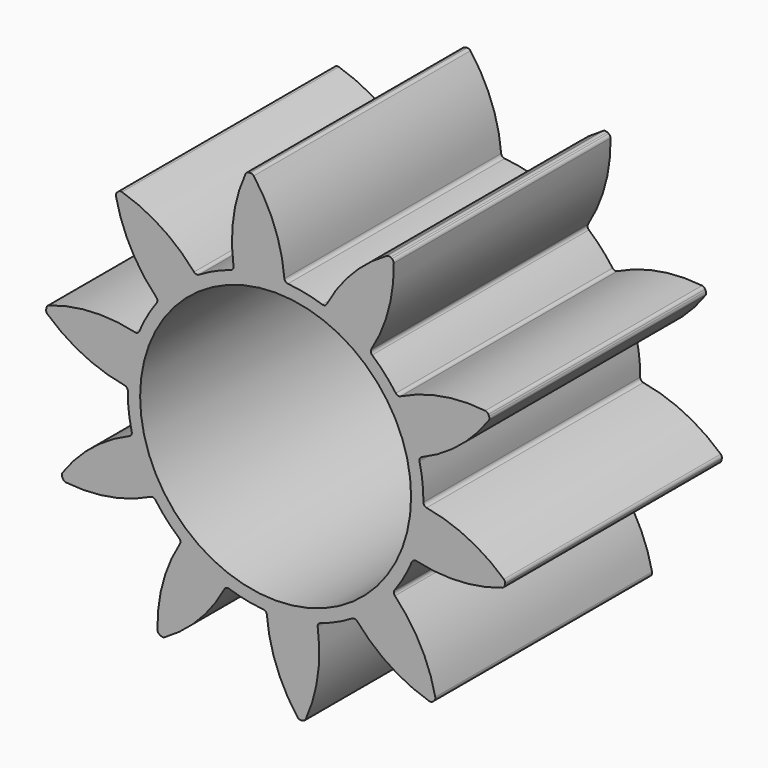
from build123d import *

# Parameters (mm, degrees)
F1_DEPTH = 2.2
F2_R     = 1.1
F3_DEPTH = 2.201


# Not quite as in the source:
# - a feature names something its author has since deleted; it is built from what else it names


with BuildPart() as f1:
    # F0 (on Front) → F1 (new body)
    with BuildSketch(Plane.XZ):
        with BuildLine():
            ThreePointArc((0.0712355079, 1.2242322703), (-0.0067892224, 1.5682114478), (-0.1777987566, 1.8767001385))
            ThreePointArc((-0.1777987566, 1.8767001385), (-0.1902412648, 1.886460015), (-0.2058788954, 1.888812823))
            ThreePointArc((-0.2058788954, 1.888812823), (-0.2127325046, 1.8880531988), (-0.2195833118, 1.8872687061))
            ThreePointArc((-0.2195833118, 1.8872687061), (-0.2343053253, 1.8814951877), (-0.244264097, 1.8692112932))
            ThreePointArc((-0.244264097, 1.8692112932), (-0.3423408736, 1.5304038568), (-0.3418667931, 1.1776868196))
            ThreePointArc((-0.3418667931, 1.1776868196), (-0.3462894397, 1.1567994489), (-0.3631689361, 1.1437256331))
            ThreePointArc((-0.3631689361, 1.1437256331), (-0.496270206, 1.092573056), (-0.6223642321, 1.025993549))
            ThreePointArc((-0.6223642321, 1.025993549), (-0.8096046551, 0.885742797), (-0.966074901, 0.7118281293))
            ThreePointArc((-0.966074901, 0.7118281293), (-1.0436893598, 0.5922098617), (-1.1065671175, 0.4642297001))
            ThreePointArc((-1.1065671175, 0.4642297001), (-1.1756104781, 0.2407072989), (-1.1999730893, 0.0080364743))
            ThreePointArc((-1.1999730893, 0.0080364743), (-1.1924546519, -0.1343573713), (-1.1680989749, -0.2748541157))
            ThreePointArc((-1.1680989749, -0.2748541157), (-1.092573056, -0.496270206), (-0.9755223431, -0.6988248408))
            ThreePointArc((-0.9755223431, -0.6988248408), (-0.885742797, -0.8096046551), (-0.7834567261, -0.9089530012))
            ThreePointArc((-0.7834567261, -0.9089530012), (-0.5922098617, -1.0436893598), (-0.3784552187, -1.1387588188))
            ThreePointArc((-0.3784552187, -1.1387588188), (-0.2407072989, -1.1756104781), (-0.0995606366, -1.1958627344))
            ThreePointArc((-0.0995606366, -1.1958627344), (0.1343573713, -1.1924546519), (0.3631689361, -1.1437256331))
            ThreePointArc((0.3631689361, -1.1437256331), (0.496270206, -1.092573056), (0.6223642321, -1.025993549))
            ThreePointArc((0.6223642321, -1.025993549), (0.8096046551, -0.885742797), (0.966074901, -0.7118281293))
            ThreePointArc((0.966074901, -0.7118281293), (1.0436893598, -0.5922098617), (1.1065671175, -0.4642297001))
            ThreePointArc((1.1065671175, -0.4642297001), (1.1756104781, -0.2407072989), (1.1999730893, -0.0080364743))
            ThreePointArc((1.1999730893, -0.0080364743), (1.1924546519, 0.1343573713), (1.1680989749, 0.2748541157))
            ThreePointArc((1.1680989749, 0.2748541157), (1.092573056, 0.496270206), (0.9755223431, 0.6988248408))
            ThreePointArc((0.9755223431, 0.6988248408), (0.885742797, 0.8096046551), (0.7834567261, 0.9089530012))
            ThreePointArc((0.7834567261, 0.9089530012), (0.5922098617, 1.0436893598), (0.3784552187, 1.1387588188))
            ThreePointArc((0.3784552187, 1.1387588188), (0.2407072989, 1.1756104781), (0.0995606366, 1.1958627344))
            ThreePointArc((0.0995606366, 1.1958627344), (0.0801951467, 1.2048527211), (0.0712355079, 1.2242322703))
        make_face()
        with BuildLine():
            ThreePointArc((-0.966074901, 0.7118281293), (-0.8096046551, 0.885742797), (-0.6223642321, 1.025993549))
            ThreePointArc((-0.6223642321, 1.025993549), (-0.6433154241, 1.0218838516), (-0.6619549374, 1.0322958927))
            ThreePointArc((-0.6619549374, 1.0322958927), (-0.9272641578, 1.2647191073), (-1.2469388801, 1.4137748184))
            ThreePointArc((-1.2469388801, 1.4137748184), (-1.262741792, 1.4143572015), (-1.2767758469, 1.4070690946))
            ThreePointArc((-1.2767758469, 1.4070690946), (-1.2818740373, 1.4024260952), (-1.2869553435, 1.3977646239))
            ThreePointArc((-1.2869553435, 1.3977646239), (-1.2954721137, 1.3844403669), (-1.2963086372, 1.3686488684))
            ThreePointArc((-1.2963086372, 1.3686488684), (-1.1765084017, 1.0368998116), (-0.9688029898, 0.7518243919))
            ThreePointArc((-0.9688029898, 0.7518243919), (-0.9601036976, 0.7323265875), (-0.966074901, 0.7118281293))
        make_face()
        with BuildLine():
            ThreePointArc((-0.9755223431, -0.6988248408), (-1.092573056, -0.496270206), (-1.1680989749, -0.2748541157))
            ThreePointArc((-1.1680989749, -0.2748541157), (-1.1706646948, -0.2960498497), (-1.1863270607, -0.3105595826))
            ThreePointArc((-1.1863270607, -0.3105595826), (-1.4893597313, -0.4910609223), (-1.7299050585, -0.7490289022))
            ThreePointArc((-1.7299050585, -0.7490289022), (-1.7353423061, -0.7638783983), (-1.7327476659, -0.7794777265))
            ThreePointArc((-1.7327476659, -0.7794777265), (-1.7299073387, -0.7857611594), (-1.7270442259, -0.7920342427))
            ThreePointArc((-1.7270442259, -0.7920342427), (-1.7170039312, -0.8042515943), (-1.7022438237, -0.8099270169))
            ThreePointArc((-1.7022438237, -0.8099270169), (-1.3497114128, -0.7985063187), (-1.0144040751, -0.6890598826))
            ThreePointArc((-1.0144040751, -0.6890598826), (-0.9931723321, -0.686811517), (-0.9755223431, -0.6988248408))
        make_face()
        with BuildLine():
            ThreePointArc((0.3418667931, -1.1776868196), (0.3462894397, -1.1567994489), (0.3631689361, -1.1437256331))
            ThreePointArc((0.3631689361, -1.1437256331), (0.1343573713, -1.1924546519), (-0.0995606366, -1.1958627344))
            ThreePointArc((-0.0995606366, -1.1958627344), (-0.0801951467, -1.2048527211), (-0.0712355079, -1.2242322703))
            ThreePointArc((-0.0712355079, -1.2242322703), (0.0067892224, -1.5682114478), (0.1777987566, -1.8767001385))
            ThreePointArc((0.1777987566, -1.8767001385), (0.1902412648, -1.886460015), (0.2058788954, -1.888812823))
            ThreePointArc((0.2058788954, -1.888812823), (0.2127325046, -1.8880531988), (0.2195833118, -1.8872687061))
            ThreePointArc((0.2195833118, -1.8872687061), (0.2343053253, -1.8814951877), (0.244264097, -1.8692112932))
            ThreePointArc((0.244264097, -1.8692112932), (0.3423408736, -1.5304038568), (0.3418667931, -1.1776868196))
        make_face()
        with BuildLine():
            ThreePointArc((0.9688029898, -0.7518243919), (0.9601036976, -0.7323265875), (0.966074901, -0.7118281293))
            ThreePointArc((0.966074901, -0.7118281293), (0.8096046551, -0.885742797), (0.6223642321, -1.025993549))
            ThreePointArc((0.6223642321, -1.025993549), (0.6433154241, -1.0218838516), (0.6619549374, -1.0322958927))
            ThreePointArc((0.6619549374, -1.0322958927), (0.9272641578, -1.2647191073), (1.2469388801, -1.4137748184))
            ThreePointArc((1.2469388801, -1.4137748184), (1.262741792, -1.4143572015), (1.2767758469, -1.4070690946))
            ThreePointArc((1.2767758469, -1.4070690946), (1.2818740373, -1.4024260952), (1.2869553435, -1.3977646239))
            ThreePointArc((1.2869553435, -1.3977646239), (1.2954721137, -1.3844403669), (1.2963086372, -1.3686488684))
            ThreePointArc((1.2963086372, -1.3686488684), (1.1765084017, -1.0368998116), (0.9688029898, -0.7518243919))
        make_face()
        with BuildLine():
            ThreePointArc((1.2256893728, -0.0387906), (1.2071909758, -0.0281298606), (1.1999730893, -0.0080364743))
            ThreePointArc((1.1999730893, -0.0080364743), (1.1756104781, -0.2407072989), (1.1065671175, -0.4642297001))
            ThreePointArc((1.1065671175, -0.4642297001), (1.1211013684, -0.4485900834), (1.1423010956, -0.4460575705))
            ThreePointArc((1.1423010956, -0.4460575705), (1.4935557015, -0.478147054), (1.8397907332, -0.4108355701))
            ThreePointArc((1.8397907332, -0.4108355701), (1.8529178738, -0.4020180093), (1.8599878209, -0.3878727965))
            ThreePointArc((1.8599878209, -0.3878727965), (1.861383257, -0.38111989), (1.862754176, -0.3743619636))
            ThreePointArc((1.862754176, -0.3743619636), (1.861812586, -0.3585763814), (1.8532073379, -0.3453090945))
            ThreePointArc((1.8532073379, -0.3453090945), (1.5612897084, -0.1473352813), (1.2256893728, -0.0387906))
        make_face()
        with BuildLine():
            ThreePointArc((1.0144040751, 0.6890598826), (0.9931723321, 0.686811517), (0.9755223431, 0.6988248408))
            ThreePointArc((0.9755223431, 0.6988248408), (1.092573056, 0.496270206), (1.1680989749, 0.2748541157))
            ThreePointArc((1.1680989749, 0.2748541157), (1.1706646948, 0.2960498497), (1.1863270607, 0.3105595826))
            ThreePointArc((1.1863270607, 0.3105595826), (1.4893597313, 0.4910609223), (1.7299050585, 0.7490289022))
            ThreePointArc((1.7299050585, 0.7490289022), (1.7353423061, 0.7638783983), (1.7327476659, 0.7794777265))
            ThreePointArc((1.7327476659, 0.7794777265), (1.7299073387, 0.7857611594), (1.7270442259, 0.7920342427))
            ThreePointArc((1.7270442259, 0.7920342427), (1.7170039312, 0.8042515943), (1.7022438237, 0.8099270169))
            ThreePointArc((1.7022438237, 0.8099270169), (1.3497114128, 0.7985063187), (1.0144040751, 0.6890598826))
        make_face()
        with BuildLine():
            ThreePointArc((0.4156508989, 1.1537129104), (0.3997956142, 1.139414239), (0.3784552187, 1.1387588188))
            ThreePointArc((0.3784552187, 1.1387588188), (0.5922098617, 1.0436893598), (0.7834567261, 0.9089530012))
            ThreePointArc((0.7834567261, 0.9089530012), (0.7730738972, 0.9276088025), (0.7772164104, 0.9485535308))
            ThreePointArc((0.7772164104, 0.9485535308), (0.9162789653, 1.2727003169), (0.9592544487, 1.6227897924))
            ThreePointArc((0.9592544487, 1.6227897924), (0.9549249596, 1.6379992211), (0.9436567966, 1.6490942515))
            ThreePointArc((0.9436567966, 1.6490942515), (0.9376656143, 1.652508153), (0.9316620816, 1.6559002886))
            ThreePointArc((0.9316620816, 1.6559002886), (0.9163581335, 1.6598827965), (0.901081026, 1.6557985362))
            ThreePointArc((0.901081026, 1.6557985362), (0.6225892324, 1.4393456452), (0.4156508989, 1.1537129104))
        make_face()
        with BuildLine():
            ThreePointArc((-1.1999730893, 0.0080364743), (-1.1756104781, 0.2407072989), (-1.1065671175, 0.4642297001))
            ThreePointArc((-1.1065671175, 0.4642297001), (-1.1211013684, 0.4485900834), (-1.1423010956, 0.4460575705))
            ThreePointArc((-1.1423010956, 0.4460575705), (-1.4935557015, 0.478147054), (-1.8397907332, 0.4108355701))
            ThreePointArc((-1.8397907332, 0.4108355701), (-1.8529178738, 0.4020180093), (-1.8599878209, 0.3878727965))
            ThreePointArc((-1.8599878209, 0.3878727965), (-1.861383257, 0.38111989), (-1.862754176, 0.3743619636))
            ThreePointArc((-1.862754176, 0.3743619636), (-1.861812586, 0.3585763814), (-1.8532073379, 0.3453090945))
            ThreePointArc((-1.8532073379, 0.3453090945), (-1.5612897084, 0.1473352813), (-1.2256893728, 0.0387906))
            ThreePointArc((-1.2256893728, 0.0387906), (-1.2071909758, 0.0281298606), (-1.1999730893, 0.0080364743))
        make_face()
        with BuildLine():
            ThreePointArc((-0.3784552187, -1.1387588188), (-0.5922098617, -1.0436893598), (-0.7834567261, -0.9089530012))
            ThreePointArc((-0.7834567261, -0.9089530012), (-0.7730738972, -0.9276088025), (-0.7772164104, -0.9485535308))
            ThreePointArc((-0.7772164104, -0.9485535308), (-0.9162789653, -1.2727003169), (-0.9592544487, -1.6227897924))
            ThreePointArc((-0.9592544487, -1.6227897924), (-0.9549249596, -1.6379992211), (-0.9436567966, -1.6490942515))
            ThreePointArc((-0.9436567966, -1.6490942515), (-0.9376656143, -1.652508153), (-0.9316620816, -1.6559002886))
            ThreePointArc((-0.9316620816, -1.6559002886), (-0.9163581335, -1.6598827965), (-0.901081026, -1.6557985362))
            ThreePointArc((-0.901081026, -1.6557985362), (-0.6225892324, -1.4393456452), (-0.4156508989, -1.1537129104))
            ThreePointArc((-0.4156508989, -1.1537129104), (-0.3997956142, -1.139414239), (-0.3784552187, -1.1387588188))
        make_face()
    extrude(amount=F1_DEPTH)

    # F2 (on face) → F3 (cut, through all)
    with BuildSketch(Plane.XZ.offset(2.2)):
        Circle(F2_R)
    extrude(amount=-F3_DEPTH, mode=Mode.SUBTRACT)


solid = f1.part
